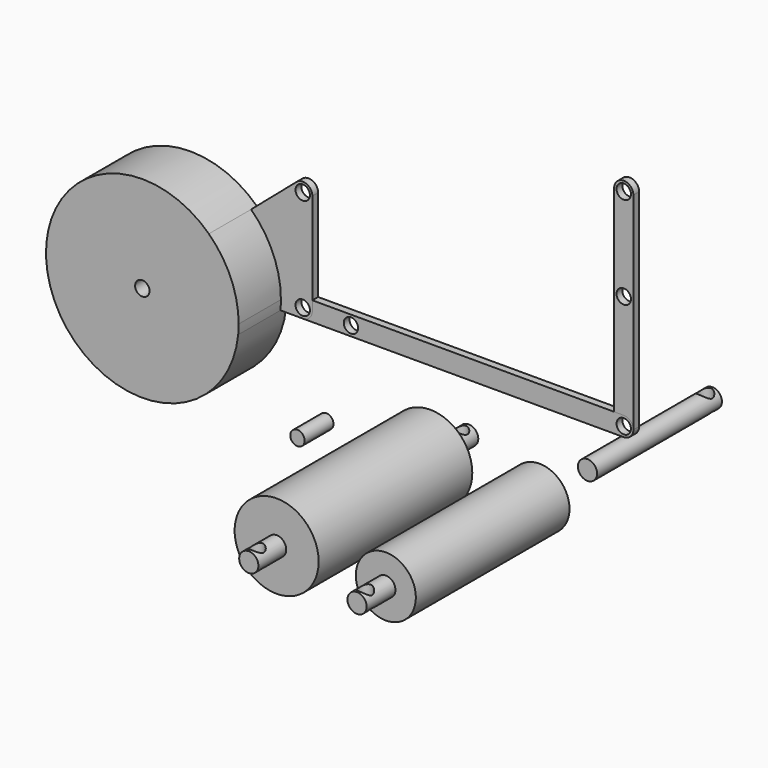
from build123d import *

# Parameters (mm, degrees)
F0_R      = 4
F1_DEPTH  = 65
F0_R_2    = 17.5
F2_DEPTH  = 80
F3_R      = 4
F4_DEPTH  = 20
F5_R      = 2.7212500561
F6_DEPTH  = 57.1348365972
F7_R      = 4
F8_DEPTH  = 14.5
F9_R      = 3
F10_DEPTH = 57.1348365972
F0_R_3    = 3
F11_DEPTH = 15
F0_R_4    = 12.5
F12_DEPTH = 80
F13_R     = 4
F14_DEPTH = 15
F15_R     = 3
F16_DEPTH = 57.1348365972
F17_START = -25
F17_DEPTH = 65
F18_R     = 3
F19_DEPTH = 57.1348365972
F20_DEPTH = 3
F21_DEPTH = 3
F22_DEPTH = 3
F23_DEPTH = 25


with BuildPart() as f1:
    # F0 (on Front) → F1 (new body)
    with BuildSketch(Plane.XZ):
        with Locations((50.7327988744, -39.6338365972)):
            Circle(F0_R)
    extrude(amount=F1_DEPTH)

    # F3 (on face) → F4 (join)
    with BuildSketch(Plane(origin=(0, 0, 0), x_dir=(-1, 0, 0), z_dir=(0, 1, 0))):
        with Locations((-50.7327988744, -39.6338365972)):
            Circle(F3_R)
    extrude(amount=F4_DEPTH)

    # F5 (on Top) → F6 (cut, through all)
    with BuildSketch(Plane.XY):
        with Locations((50.7936961949, 15.8873330802)):
            Circle(F5_R)
    extrude(amount=-F6_DEPTH, mode=Mode.SUBTRACT)


with BuildPart() as f2:
    # F0 (on Front) → F2 (new body)
    with BuildSketch(Plane.XZ):
        with Locations((50.7327988744, -39.6338365972)):
            Circle(F0_R_2)
        with Locations((50.7327988744, -39.6338365972)):
            Circle(F0_R, mode=Mode.SUBTRACT)
    extrude(amount=F2_DEPTH)


with BuildPart() as f8:
    # F7 (on face) → F8 (new body)
    with BuildSketch(Plane.XZ.offset(80)):
        with Locations((50.7327988744, -39.6338365972)):
            Circle(F7_R)
    extrude(amount=F8_DEPTH)

    # F9 (on Top) → F10 (cut, through all)
    with BuildSketch(Plane.XY):
        with Locations((50.6241805851, -90.323202312)):
            Circle(F9_R)
    extrude(amount=-F10_DEPTH, mode=Mode.SUBTRACT)


with BuildPart() as f11:
    # F0 (on Front) → F11 (new body)
    with BuildSketch(Plane.XZ):
        with Locations((7.40870554, -40.5091047287)):
            Circle(F0_R_3)
    extrude(amount=F11_DEPTH)


with BuildPart() as f12:
    # F0 (on Front) → F12 (new body)
    with BuildSketch(Plane.XZ):
        with Locations((96.2205678225, -39.6338365972)):
            Circle(F0_R_4)
        with Locations((96.2205678225, -39.6338365972)):
            Circle(F0_R, mode=Mode.SUBTRACT)
    extrude(amount=F12_DEPTH)


with BuildPart() as f14:
    # F13 (on face) → F14 (new body)
    with BuildSketch(Plane.XZ.offset(80)):
        with Locations((96.2205678225, -39.6338365972)):
            Circle(F13_R)
    extrude(amount=F14_DEPTH)

    # F15 (on Top) → F16 (cut, through all)
    with BuildSketch(Plane.XY):
        with Locations((96.4334607124, -91.1051779985)):
            Circle(F15_R)
    extrude(amount=-F16_DEPTH, mode=Mode.SUBTRACT)


with BuildPart() as f17:
    # F0 (on Front) → F17 (new body)
    with BuildSketch(Plane.XZ.offset(F17_START)):
        with Locations((96.2205678225, -39.6338365972)):
            Circle(F0_R)
    extrude(amount=-F17_DEPTH)

    # F18 (on Top) → F19 (cut, through all)
    with BuildSketch(Plane.XY):
        with Locations((96.3697656989, 86.0765725374)):
            Circle(F18_R)
    extrude(amount=-F19_DEPTH, mode=Mode.SUBTRACT)


with BuildPart() as f20:
    # F0 (on Front) → F20 (new body)
    with BuildSketch(Plane.XZ):
        with BuildLine():
            ThreePointArc((129.726760745, 0), (130.8983336203, -2.8284271247), (133.726760745, -4))
            ThreePointArc((133.726760745, -4), (136.5551878698, -2.8284271247), (137.726760745, 0))
            ThreePointArc((137.726760745, 0), (136.5551878698, 2.8284271247), (133.726760745, 4))
            ThreePointArc((133.726760745, 4), (130.8983336203, 2.8284271247), (129.726760745, 0))
        make_face()
        with Locations((133.726760745, 0)):
            Circle(F0_R_3, mode=Mode.SUBTRACT)
        with BuildLine():
            Line((129.726760745, 86.0603302717), (129.726760745, 4))
            Line((129.726760745, 4), (133.726760745, 4))
            ThreePointArc((133.726760745, 4), (136.5551878698, 2.8284271247), (137.726760745, 0))
            Line((137.726760745, 0), (137.726760745, 86.0603302717))
            ThreePointArc((137.726760745, 86.0603302717), (133.726760745, 82.0603302717), (129.726760745, 86.0603302717))
        make_face()
        with Locations((133.726760745, 47.5859381258)):
            Circle(F0_R_3, mode=Mode.SUBTRACT)
        with BuildLine():
            Line((133.726760745, 4), (129.726760745, 4))
            Line((129.726760745, 4), (129.726760745, 0))
            ThreePointArc((129.726760745, 0), (130.8983336203, 2.8284271247), (133.726760745, 4))
        make_face()
        with BuildLine():
            ThreePointArc((137.726760745, 86.0603302717), (133.726760745, 90.0603302717), (129.726760745, 86.0603302717))
            ThreePointArc((129.726760745, 86.0603302717), (133.726760745, 82.0603302717), (137.726760745, 86.0603302717))
        make_face()
        with Locations((133.726760745, 86.0603302717)):
            Circle(F0_R_3, mode=Mode.SUBTRACT)
    extrude(amount=F20_DEPTH)


with BuildPart() as f21:
    # F0 (on Front) → F21 (new body)
    with BuildSketch(Plane.XZ):
        with BuildLine():
            ThreePointArc((129.726760745, 0), (130.8983336203, -2.8284271247), (133.726760745, -4))
            ThreePointArc((133.726760745, -4), (136.5551878698, -2.8284271247), (137.726760745, 0))
            ThreePointArc((137.726760745, 0), (136.5551878698, 2.8284271247), (133.726760745, 4))
            ThreePointArc((133.726760745, 4), (130.8983336203, 2.8284271247), (129.726760745, 0))
        make_face()
        with Locations((133.726760745, 0)):
            Circle(F0_R_3, mode=Mode.SUBTRACT)
        with BuildLine():
            Line((133.726760745, 4), (129.726760745, 4))
            Line((129.726760745, 4), (129.726760745, 0))
            ThreePointArc((129.726760745, 0), (130.8983336203, 2.8284271247), (133.726760745, 4))
        make_face()
        with BuildLine():
            Line((4, 4), (4, 0))
            ThreePointArc((4, 0), (2.8284271247, -2.8284271247), (0, -4))
            Line((0, -4), (133.726760745, -4))
            ThreePointArc((133.726760745, -4), (130.8983336203, -2.8284271247), (129.726760745, 0))
            Line((129.726760745, 0), (129.726760745, 4))
            Line((129.726760745, 4), (4, 4))
        make_face()
        with Locations((20.0851336122, 0)):
            Circle(F0_R_3, mode=Mode.SUBTRACT)
        with BuildLine():
            ThreePointArc((0, 4), (2.8284271247, 2.8284271247), (4, 0))
            Line((4, 0), (4, 4))
            Line((4, 4), (0, 4))
        make_face()
        with BuildLine():
            ThreePointArc((0, -4), (2.8284271247, -2.8284271247), (4, 0))
            ThreePointArc((4, 0), (2.8284271247, 2.8284271247), (0, 4))
            ThreePointArc((0, 4), (-4, 0), (0, -4))
        make_face()
        Circle(F0_R_3, mode=Mode.SUBTRACT)
    extrude(amount=F21_DEPTH)


with BuildPart() as f22:
    # F0 (on Front) → F22 (new body)
    with BuildSketch(Plane.XZ):
        with BuildLine():
            ThreePointArc((0, -4), (-4, 0), (0, 4))
            Line((0, 4), (4, 4))
            Line((4, 4), (4, 42.2269292176))
            ThreePointArc((4, 42.2269292176), (-1.5626198278, 38.5447804871), (-2.7791096368, 45.1038285253))
            Line((-2.7791096368, 45.1038285253), (-21.5150295914, 29.0329656681))
            ThreePointArc((-21.5150295914, 29.0329656681), (-12.32595382, 15.790211607), (-9.088846151, 0))
            ThreePointArc((-9.088846151, 0), (-9.1388398448, -2.0024947008), (-9.2886963621, -4))
            Line((-9.2886963621, -4), (0, -4))
        make_face()
        with BuildLine():
            Line((-49.2187514901, -4), (-9.2886963621, -4))
            ThreePointArc((-9.2886963621, -4), (-9.1388398448, -2.0024947008), (-9.088846151, 0))
            ThreePointArc((-9.088846151, 0), (-12.32595382, 15.790211607), (-21.5150295914, 29.0329656681))
            Line((-21.5150295914, 29.0329656681), (-51.8229913698, 3.0361051775))
            ThreePointArc((-51.8229913698, 3.0361051775), (-47.5479671711, 3.634347226), (-45.2187514901, 0))
            ThreePointArc((-45.2187514901, 0), (-46.3903243654, -2.8284271247), (-49.2187514901, -4))
        make_face()
        with BuildLine():
            ThreePointArc((-51.8229913698, 3.0361051775), (-52.9700459807, -1.3884486468), (-49.2187514901, -4))
            ThreePointArc((-49.2187514901, -4), (-46.3903243654, -2.8284271247), (-45.2187514901, 0))
            ThreePointArc((-45.2187514901, 0), (-47.5479671711, 3.634347226), (-51.8229913698, 3.0361051775))
        make_face()
        with Locations((-49.2187514901, 0)):
            Circle(F0_R_3, mode=Mode.SUBTRACT)
        with BuildLine():
            ThreePointArc((0, -4), (2.8284271247, -2.8284271247), (4, 0))
            ThreePointArc((4, 0), (2.8284271247, 2.8284271247), (0, 4))
            ThreePointArc((0, 4), (-4, 0), (0, -4))
        make_face()
        Circle(F0_R_3, mode=Mode.SUBTRACT)
        with BuildLine():
            ThreePointArc((0, 4), (2.8284271247, 2.8284271247), (4, 0))
            Line((4, 0), (4, 4))
            Line((4, 4), (0, 4))
        make_face()
        with BuildLine():
            ThreePointArc((-2.7791096368, 45.1038285253), (-1.5626198278, 38.5447804871), (4, 42.2269292176))
            ThreePointArc((4, 42.2269292176), (1.5626198278, 45.9090779481), (-2.7791096368, 45.1038285253))
        make_face()
        with Locations((0, 42.2269292176)):
            Circle(F0_R_3, mode=Mode.SUBTRACT)
    extrude(amount=F22_DEPTH)


with BuildPart() as f23:
    # F0 (on Front) → F23 (new body)
    with BuildSketch(Plane.XZ):
        with BuildLine():
            ThreePointArc((-21.5150295914, 29.0329656681), (-86.8535246917, -13.9295781915), (-9.2886963621, -4))
            Line((-9.2886963621, -4), (-49.2187514901, -4))
            ThreePointArc((-49.2187514901, -4), (-52.9700459807, -1.3884486468), (-51.8229913698, 3.0361051775))
            Line((-51.8229913698, 3.0361051775), (-21.5150295914, 29.0329656681))
        make_face()
        with BuildLine():
            Line((-49.2187514901, -4), (-9.2886963621, -4))
            ThreePointArc((-9.2886963621, -4), (-9.1388398448, -2.0024947008), (-9.088846151, 0))
            ThreePointArc((-9.088846151, 0), (-12.32595382, 15.790211607), (-21.5150295914, 29.0329656681))
            Line((-21.5150295914, 29.0329656681), (-51.8229913698, 3.0361051775))
            ThreePointArc((-51.8229913698, 3.0361051775), (-47.5479671711, 3.634347226), (-45.2187514901, 0))
            ThreePointArc((-45.2187514901, 0), (-46.3903243654, -2.8284271247), (-49.2187514901, -4))
        make_face()
        with BuildLine():
            ThreePointArc((-51.8229913698, 3.0361051775), (-52.9700459807, -1.3884486468), (-49.2187514901, -4))
            ThreePointArc((-49.2187514901, -4), (-46.3903243654, -2.8284271247), (-45.2187514901, 0))
            ThreePointArc((-45.2187514901, 0), (-47.5479671711, 3.634347226), (-51.8229913698, 3.0361051775))
        make_face()
        with Locations((-49.2187514901, 0)):
            Circle(F0_R_3, mode=Mode.SUBTRACT)
    extrude(amount=F23_DEPTH)


solid = Compound([f1.part, f2.part, f8.part, f11.part, f12.part, f14.part, f17.part, f20.part, f21.part, f22.part, f23.part])
